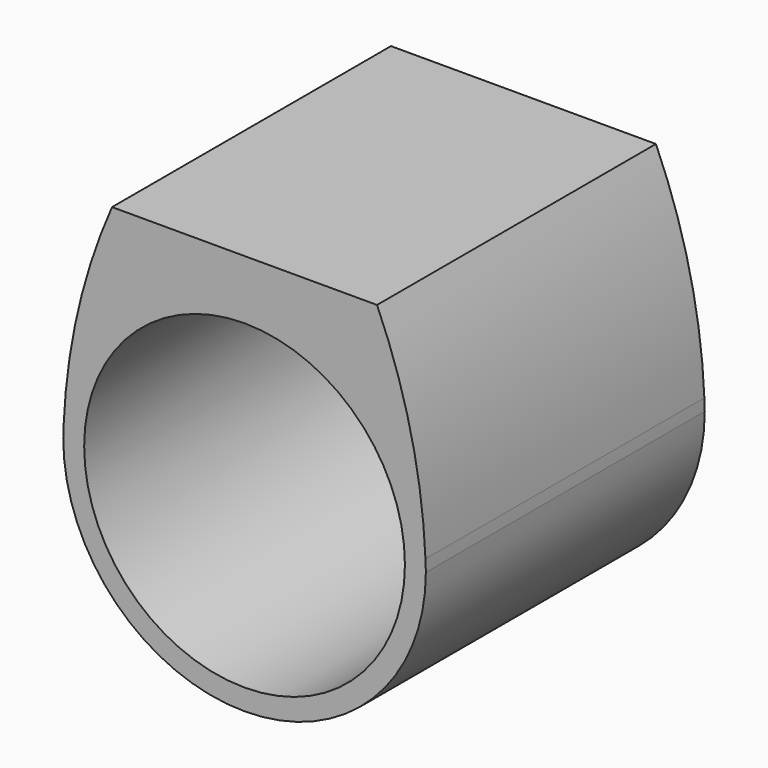
from build123d import *

# Parameters (mm, degrees)
F1_DEPTH = 25


with BuildPart() as f1:
    # F0 (on Front) → F1 (new body)
    with BuildSketch(Plane.XZ):
        with BuildLine():
            ThreePointArc((9.5, 6.4807406984), (10.9886304879, 3.3911649916), (11.5, 0))
            ThreePointArc((11.5, 0), (-3.3911649916, -10.9886304879), (-9.5, 6.4807406984))
            Line((-9.5, 6.4807406984), (-9.5, 8.8741196746))
            ThreePointArc((-9.5, 8.8741196746), (-11.932192643, 5.1597266138), (-12.9726060851, 0.8434994728))
            ThreePointArc((-12.9726060851, 0.8434994728), (-12.9884576775, 0.4218197114), (-13, 0))
            ThreePointArc((-13, 0), (0, -13), (13, 0))
            ThreePointArc((13, 0), (12.9884576775, 0.4218197114), (12.9726060851, 0.8434994728))
            ThreePointArc((12.9726060851, 0.8434994728), (11.932192643, 5.1597266138), (9.5, 8.8741196746))
            Line((9.5, 8.8741196746), (9.5, 6.4807406984))
        make_face()
        with BuildLine():
            ThreePointArc((-9.5, 6.4807406984), (0, 11.5), (9.5, 6.4807406984))
            Line((9.5, 6.4807406984), (9.5, 8.8741196746))
            ThreePointArc((9.5, 8.8741196746), (0, 13), (-9.5, 8.8741196746))
            Line((-9.5, 8.8741196746), (-9.5, 6.4807406984))
        make_face()
        with BuildLine():
            Line((9.5, 15.7431904227), (9.5, 8.8741196746))
            ThreePointArc((9.5, 8.8741196746), (11.932192643, 5.1597266138), (12.9726060851, 0.8434994728))
            ThreePointArc((12.9726060851, 0.8434994728), (11.932253156, 8.45554701), (9.5, 15.7431904227))
        make_face()
        with BuildLine():
            ThreePointArc((-9.5, 8.8741196746), (0, 13), (9.5, 8.8741196746))
            Line((9.5, 8.8741196746), (9.5, 15.7431904227))
            Line((9.5, 15.7431904227), (-9.5, 15.7431904227))
            Line((-9.5, 15.7431904227), (-9.5, 8.8741196746))
        make_face()
        with BuildLine():
            ThreePointArc((-12.9726060851, 0.8434994728), (-11.932192643, 5.1597266138), (-9.5, 8.8741196746))
            Line((-9.5, 8.8741196746), (-9.5, 15.7431904227))
            ThreePointArc((-9.5, 15.7431904227), (-11.932253156, 8.45554701), (-12.9726060851, 0.8434994728))
        make_face()
    extrude(amount=F1_DEPTH)


solid = f1.part
